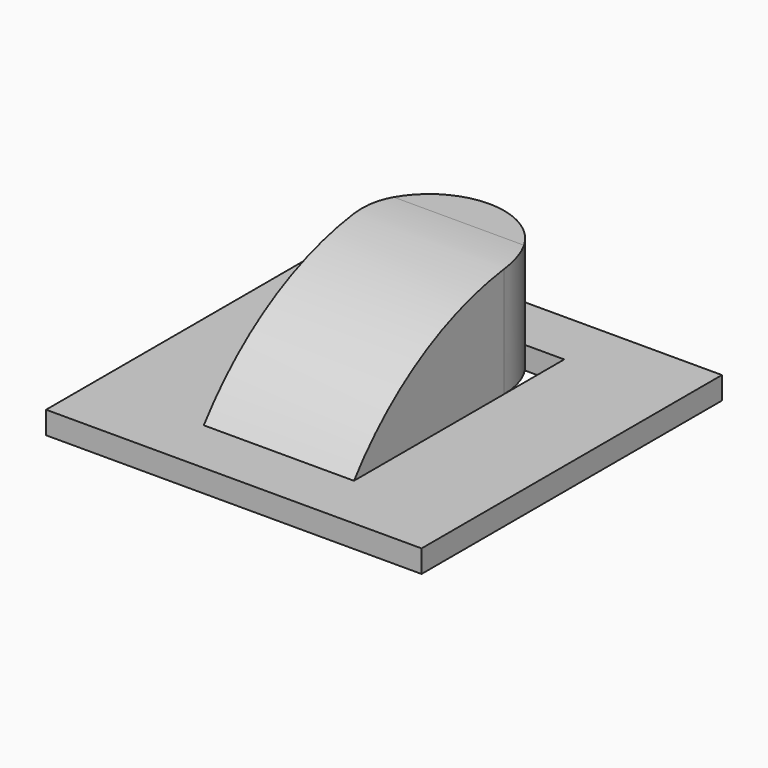
from build123d import *

# Parameters (mm, degrees)
F0_W        = 10.16
F0_H        = 17.78
F1_DEPTH    = 7.62
F2_T1_DEPTH = 86.2587266768
F3_R        = 5.07999
F0_W_2      = 25.4
F0_H_2      = 25.4
F4_DEPTH    = 1.524


# Not quite as in the source:
# - a fillet or chamfer that OpenCascade refuses, or shapes differently, is made with other operations: its cross-section is extruded or revolved along the edge and cut away or added
# - a fillet or chamfer is up to 0.001 mm smaller than in the source, because OpenCascade refuses the exact size


with BuildPart() as f1:
    # F0 (on Top) → F1 (new body)
    with BuildSketch(Plane.XY):
        with Locations((-12.7, 12.7)):
            Rectangle(F0_W, F0_H)
    extrude(amount=F1_DEPTH)

    # F2: fillet of radius 19.0095175901 on 1 edges, made by hand

    # F2_s2 → F2_t1 (cut)
    with BuildSketch(Plane.YZ.offset(-55.8293633384)):
        with BuildLine():
            ThreePointArc((3.81, 0), (10.5193832973, 5.6085851567), (19.0297453354, 7.62))
            Line((19.0297453354, 7.62), (3.81, 7.62))
            Line((3.81, 7.62), (3.81, 0))
        make_face()
    extrude(amount=F2_T1_DEPTH, mode=Mode.SUBTRACT)

    # F3 (radius 5.08 in the source; OpenCascade refuses exactly that, so slightly less here)
    f3_edges = [f1.edges().sort_by_distance(p)[0] for p in [
        (-17.78, 21.59, 3.81),
        (-7.62, 21.59, 3.81),
    ]]
    fillet(f3_edges, radius=F3_R)


with BuildPart() as f4:
    # F0 (on Top) → F4 (new body)
    with BuildSketch(Plane.XY):
        with Locations((-12.7, 12.7)):
            Rectangle(F0_W_2, F0_H_2)
        with Locations((-12.7, 12.7)):
            Rectangle(F0_W, F0_H, mode=Mode.SUBTRACT)
    extrude(amount=-F4_DEPTH)


solid = Compound([f1.part, f4.part])
